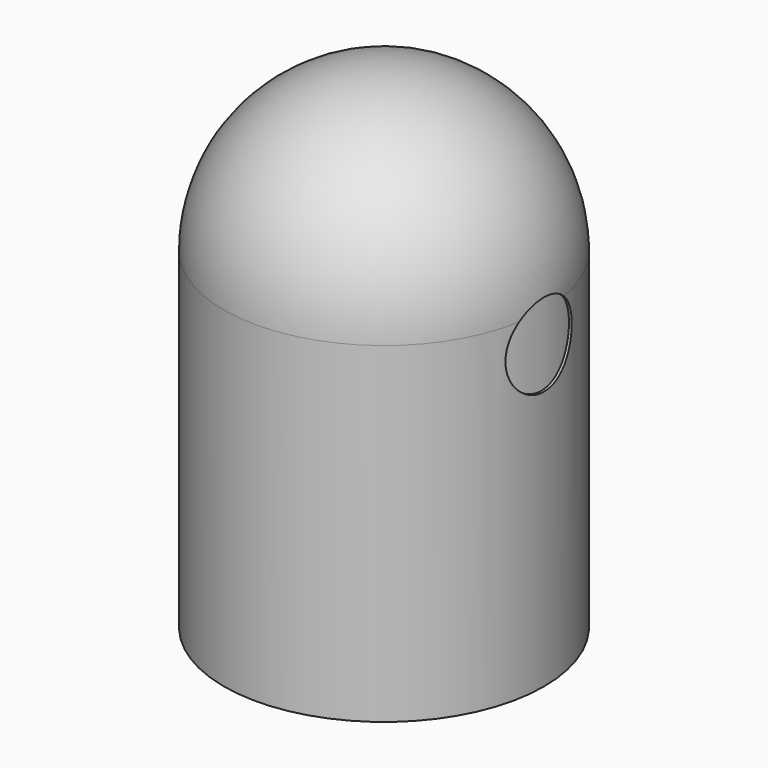
from build123d import *

# Parameters (mm, degrees)
F0_R      = 48.3
F0_R_2    = 47.5
F1_DEPTH  = 100
F3_ANGLE  = 180
F5_R      = 12.5
F6_DEPTH  = 6
F9_R      = 12.5
F10_DEPTH = 6


with BuildPart() as f1:
    # F0 (on Top) → F1 (new body)
    with BuildSketch(Plane.XY):
        Circle(F0_R)
        Circle(F0_R_2, mode=Mode.SUBTRACT)
    extrude(amount=F1_DEPTH)

    # F2 (on face) → F3 (revolve)
    with BuildSketch(Plane.XY.offset(100)):
        with BuildLine():
            ThreePointArc((47.5, 0), (0, -47.5), (-47.5, 0))
            Line((-47.5, 0), (-48.3, 0))
            ThreePointArc((-48.3, 0), (0, -48.3), (48.3, 0))
            Line((48.3, 0), (47.5, 0))
        make_face()
    revolve(axis=Axis((-47.9, 0, 100), (-1, 0, 0)), revolution_arc=F3_ANGLE)

    # F5 (on offset) → F6 (cut)
    with BuildSketch(Plane.YZ.offset(49)):
        with Locations((0, 90.8108726144)):
            Circle(F5_R)
    extrude(amount=-F6_DEPTH, mode=Mode.SUBTRACT)

    # F9 (on face) → F10 (cut)
    with BuildSketch(Plane(origin=(24.5, 42.4352447854, 0), x_dir=(-0.8660254038, 0.5, 0), z_dir=(0.5, 0.8660254038, 0))):
        with Locations((0, 90.4301926494)):
            Circle(F9_R)
    extrude(amount=-F10_DEPTH, mode=Mode.SUBTRACT)


solid = f1.part
